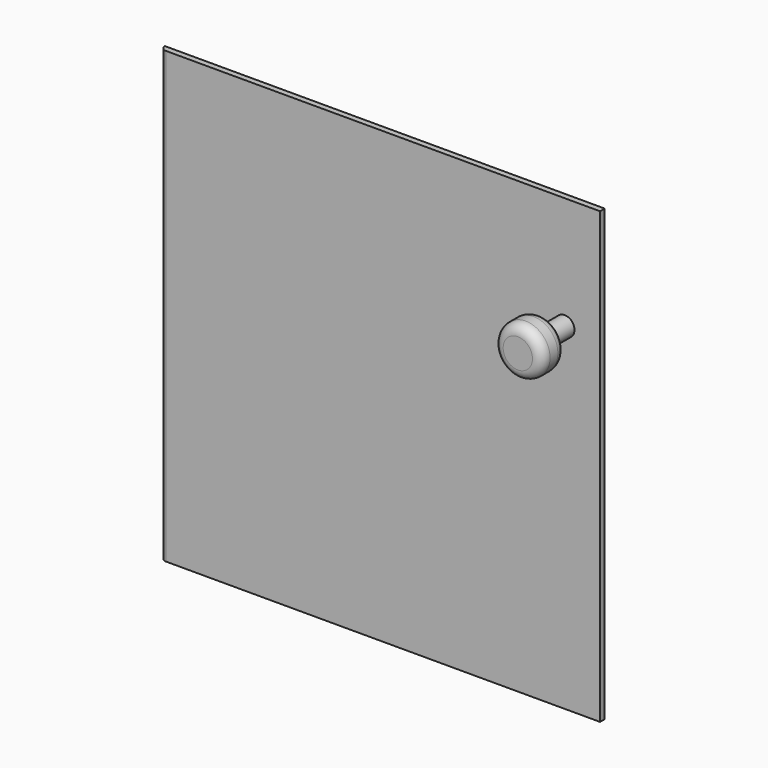
from build123d import *

# Parameters (mm, degrees)
F0_W     = 571.5
F0_H     = 584.2
F1_DEPTH = 7.62
F2_R     = 7.61999
F3_R     = 12.7
F4_DEPTH = 38.1
F5_R     = 31.75
F5_R_2   = 12.7
F6_DEPTH = 38.1
F7_R     = 12.7


# Not quite as in the source:
# - a fillet or chamfer is up to 0.001 mm smaller than in the source, because OpenCascade refuses the exact size


with BuildPart() as f1:
    # F0 (on Front) → F1 (new body)
    with BuildSketch(Plane.XZ):
        with Locations((-17.7775520504, 93.1158526728)):
            Rectangle(F0_W, F0_H)
    extrude(amount=F1_DEPTH)

    # F2 (radius 7.62 in the source; OpenCascade refuses exactly that, so slightly less here)
    f2_edges = [f1.edges().sort_by_distance(p)[0] for p in [
        (-303.527552, -7.62, 93.115853),
    ]]
    fillet(f2_edges, radius=F2_R)

    # F3 (on face) → F4 (join)
    with BuildSketch(Plane.XZ.offset(7.62)):
        with Locations((222.1034169197, 238.7578934431)):
            Circle(F3_R)
    extrude(amount=F4_DEPTH)

    # F5 (on face) → F6 (join)
    with BuildSketch(Plane.XZ.offset(45.72)):
        with Locations((222.1034169197, 238.7578934431)):
            Circle(F5_R)
        with Locations((222.1034169197, 238.7578934431)):
            Circle(F5_R_2, mode=Mode.SUBTRACT)
        with Locations((222.1034169197, 238.7578934431)):
            Circle(F5_R_2)
    extrude(amount=F6_DEPTH)

    # F7
    f7_edges = [f1.edges().sort_by_distance(p)[0] for p in [
        (190.353417, -83.82, 238.757893),
        (190.353417, -45.72, 238.757893),
    ]]
    fillet(f7_edges, radius=F7_R)


solid = f1.part
